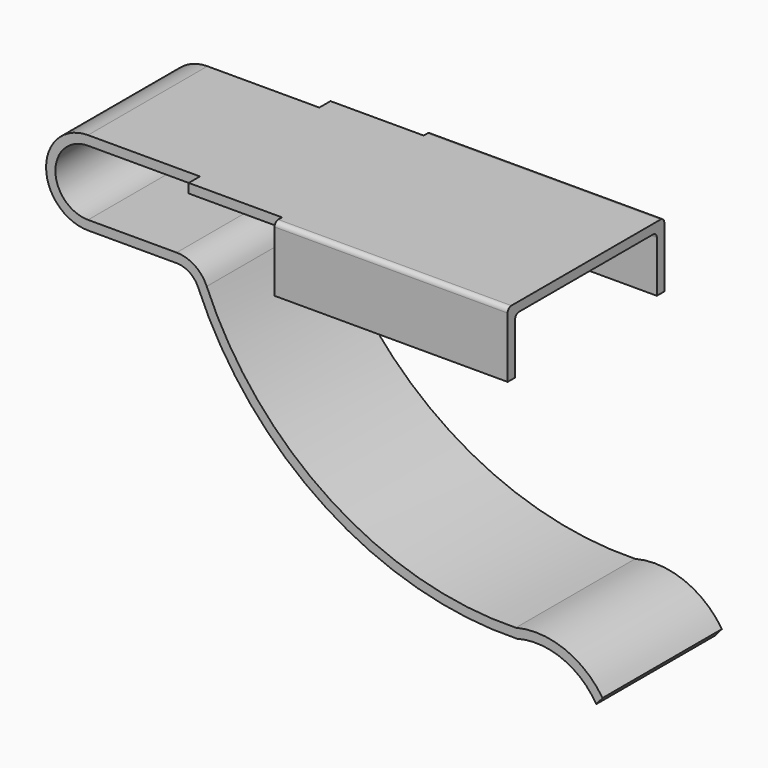
from build123d import *

# Parameters (mm, degrees)
F1_DEPTH = 16
F2_W     = 70
F2_H     = 3
F3_DEPTH = 2
F4_W     = 50
F4_H     = 14
F5_DEPTH = 2
F6_R     = 1


with BuildPart() as f1:
    # F0 (on Front) → F1 (new body)
    with BuildSketch(Plane.XZ):
        with BuildLine():
            Line((94, 18), (0, 18))
            ThreePointArc((0, 18), (-9, 9), (0, 0))
            Line((0, 0), (19, 0))
            ThreePointArc((19, 0), (21.7681124643, -0.8361612201), (23.6103896104, -3.064978646))
            ThreePointArc((23.6103896104, -3.064978646), (50.9877645087, -35.7155080232), (92.0282848079, -47.1720964556))
            ThreePointArc((92.0282848079, -47.1720964556), (101.6638981451, -47.7394028226), (109.0104486201, -54))
            Line((109.0104486201, -54), (110.3606353849, -52.3909100723))
            ThreePointArc((110.3606353849, -52.3909100723), (102.2069764649, -45.8036465806), (91.7435184361, -45.1789545189))
            ThreePointArc((91.7435184361, -45.1789545189), (51.9754606004, -33.9725556125), (25.4545454545, -2.2909701044))
            ThreePointArc((25.4545454545, -2.2909701044), (22.87535745, 0.8293742919), (19, 2))
            Line((19, 2), (0, 2))
            ThreePointArc((0, 2), (-7, 9), (0, 16))
            Line((0, 16), (94, 16))
            Line((94, 16), (94, 18))
        make_face()
    extrude(amount=F1_DEPTH)

    # F2 (on face) → F3 (join)
    with BuildSketch(Plane.XY.offset(18)):
        with Locations((59, -17.5)):
            Rectangle(F2_W, F2_H)
    extrude(amount=-F3_DEPTH)

    # F4 (on face) → F5 (join)
    with BuildSketch(Plane.XZ.offset(19)):
        with Locations((69, 11)):
            Rectangle(F4_W, F4_H)
    extrude(amount=F5_DEPTH)

    # F6
    f6_edges = [f1.edges().sort_by_distance(p)[0] for p in [
        (69, -21, 18),
        (69, -19, 16),
    ]]
    fillet(f6_edges, radius=F6_R)

    # F7: F1 across plane


with BuildPart() as f1_1:
    add(f1.part)
    add(f1.part.mirror(Plane.XZ))


solid = f1_1.part
